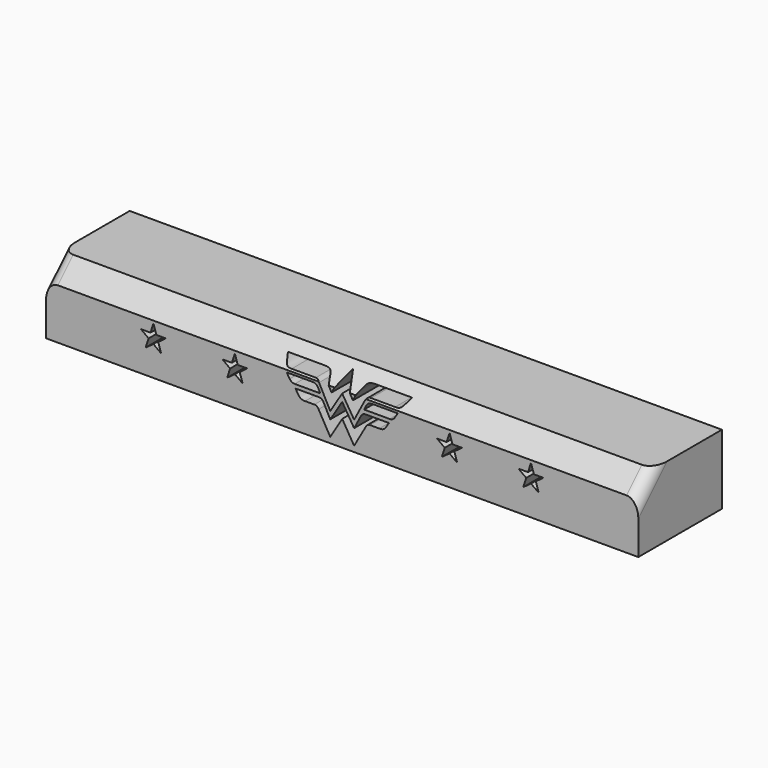
from build123d import *

# Parameters (mm, degrees)
F0_W        = 215.9
F0_H        = 25.4
F1_DEPTH    = 38.1
F3_DEPTH    = 38.1
F4_T1_DEPTH = 251.8264113419
F5_R        = 4.2924717139


# Not quite as in the source:
# - a fillet or chamfer that OpenCascade refuses, or shapes differently, is made with other operations: its cross-section is extruded or revolved along the edge and cut away or added


with BuildPart() as f1:
    # F0 (on Front) → F1 (new body)
    with BuildSketch(Plane.XZ):
        with Locations((0.6619617343, 8.3113107191)):
            Rectangle(F0_W, F0_H)
        with BuildLine():
            add(Edge.make_bspline(
                [(-16.3802020252, 9.0824095532), (-14.8727670312, 6.4565530047), (-14.5080648363, 6.1891046353), (-12.8547474742, 6.1647910625)],
                knots=[0, 0, 0, 0, 4.576169517, 4.576169517, 4.576169517, 4.576169517], degree=3))
            Line((-16.3802020252, 9.0824095532), (-8.1136170775, 9.0824095532))
            add(Edge.make_bspline(
                [(-8.1136170775, 9.0824095532), (-7.2759063914, 9.0653235093), (-6.6012172028, 8.9528746903), (-6.0469708405, 7.769481279)],
                knots=[0, 0, 0, 0, 2.4484295624, 2.4484295624, 2.4484295624, 2.4484295624], degree=3))
            Line((-6.0469708405, 7.769481279), (-3.6874657962, 3.2825956335))
            Line((-3.6874657962, 3.2825956335), (0.6619617343, 10.3273617318))
            Line((0.6619617343, 10.3273617318), (5.0113892648, 3.2825956335))
            Line((5.0113892648, 3.2825956335), (7.3708943091, 7.769481279))
            add(Edge.make_bspline(
                [(9.4375405461, 9.0824095532), (8.59982986, 9.0653235093), (7.9251406714, 8.9528746903), (7.3708943091, 7.769481279)],
                knots=[0, 0, 0, 0, 2.4484295624, 2.4484295624, 2.4484295624, 2.4484295624], degree=3))
            Line((9.4375405461, 9.0824095532), (17.7041254938, 9.0824095532))
            add(Edge.make_bspline(
                [(17.7041254938, 9.0824095532), (16.1966904998, 6.4565530047), (15.8319883049, 6.1891046353), (14.1786709428, 6.1647910625)],
                knots=[0, 0, 0, 0, 4.576169517, 4.576169517, 4.576169517, 4.576169517], degree=3))
            Line((14.1786709428, 6.1647910625), (10.7990959659, 6.1647910625))
            add(Edge.make_bspline(
                [(10.7990959659, 6.1647910625), (9.8487436771, 6.1233234592), (9.8487436771, 5.8779818937), (9.2673460022, 5.1436247304)],
                knots=[0, 0, 0, 0, 1.840934173, 1.840934173, 1.840934173, 1.840934173], degree=3))
            Line((9.2673460022, 5.1436247304), (5.0113892648, -2.3575623054))
            Line((5.0113892648, -2.3575623054), (0.6619617343, 4.8800110817))
            Line((0.6619617343, 4.8800110817), (-3.6874657962, -2.3575623054))
            Line((-3.6874657962, -2.3575623054), (-7.9434225336, 5.1436247304))
            add(Edge.make_bspline(
                [(-9.4751724973, 6.1647910625), (-8.5248202085, 6.1233234592), (-8.5248202085, 5.8779818937), (-7.9434225336, 5.1436247304)],
                knots=[0, 0, 0, 0, 1.840934173, 1.840934173, 1.840934173, 1.840934173], degree=3))
            Line((-9.4751724973, 6.1647910625), (-12.8547474742, 6.1647910625))
        make_face(mode=Mode.SUBTRACT)
        with BuildLine():
            Line((-18.4998314541, 11.4835865716), (-19.5860914445, 13.219167863))
            Line((-19.5860914445, 13.219167863), (-10.0794029066, 13.219167863))
            ThreePointArc((-10.0794029066, 13.219167863), (-8.9329270461, 12.8954335527), (-8.1251045992, 12.0198573444))
            Line((-8.1251045992, 12.0198573444), (-7.3300511576, 10.4545447975))
            Line((-7.3300511576, 10.4545447975), (-16.641804624, 10.4545447975))
            ThreePointArc((-16.641804624, 10.4545447975), (-17.7037828104, 10.7289859143), (-18.4998314541, 11.4835865716))
        make_face(mode=Mode.SUBTRACT)
        with BuildLine():
            add(Edge.make_bspline(
                [(-21.9861995429, 17.5955053419), (-19.9910327792, 14.315311797), (-19.9910327792, 14.6534768865), (-18.1987602264, 14.5858433098)],
                knots=[0, 0, 0, 0, 4.83764014, 4.83764014, 4.83764014, 4.83764014], degree=3))
            Line((-21.9861995429, 17.5955053419), (-8.4934448823, 17.5955053419))
            add(Edge.make_bspline(
                [(-8.4934448823, 17.5955053419), (-6.0586617328, 17.5616890192), (-5.8219470084, 17.1220749617), (-5.0103529356, 15.4312541708)],
                knots=[0, 0, 0, 0, 4.1007209903, 4.1007209903, 4.1007209903, 4.1007209903], degree=3))
            Line((-5.0103529356, 15.4312541708), (-3.2304712382, 12.0465927742))
            Line((-3.2304712382, 12.0465927742), (0.6619617343, 18.9819801599))
            Line((0.6619617343, 18.9819801599), (4.5543947068, 12.0465927742))
            Line((4.5543947068, 12.0465927742), (6.3342764042, 15.4312541708))
            add(Edge.make_bspline(
                [(9.8173683509, 17.5955053419), (7.3825852014, 17.5616890192), (7.145870477, 17.1220749617), (6.3342764042, 15.4312541708)],
                knots=[0, 0, 0, 0, 4.1007209903, 4.1007209903, 4.1007209903, 4.1007209903], degree=3))
            Line((9.8173683509, 17.5955053419), (23.3101230115, 17.5955053419))
            add(Edge.make_bspline(
                [(23.3101230115, 17.5955053419), (21.3149562478, 14.315311797), (21.3149562478, 14.6534768865), (19.522683695, 14.5858433098)],
                knots=[0, 0, 0, 0, 4.83764014, 4.83764014, 4.83764014, 4.83764014], degree=3))
            Line((19.522683695, 14.5858433098), (10.7304118574, 14.5858433098))
            add(Edge.make_bspline(
                [(10.7304118574, 14.5858433098), (9.9142082036, 14.5666254684), (9.6125975251, 14.456034638), (9.1072237119, 13.7742487714)],
                knots=[0, 0, 0, 0, 1.814779725, 1.814779725, 1.814779725, 1.814779725], degree=3))
            Line((9.1072237119, 13.7742487714), (5.0113892648, 5.9855217114))
            Line((5.0113892648, 5.9855217114), (0.6619617343, 13.0302878097))
            Line((0.6619617343, 13.0302878097), (-3.6874657962, 5.9855217114))
            Line((-3.6874657962, 5.9855217114), (-7.7833002433, 13.7742487714))
            add(Edge.make_bspline(
                [(-9.4064883888, 14.5858433098), (-8.590284735, 14.5666254684), (-8.2886740565, 14.456034638), (-7.7833002433, 13.7742487714)],
                knots=[0, 0, 0, 0, 1.814779725, 1.814779725, 1.814779725, 1.814779725], degree=3))
            Line((-9.4064883888, 14.5858433098), (-18.1987602264, 14.5858433098))
        make_face(mode=Mode.SUBTRACT)
        with BuildLine():
            Line((11.4033263752, 13.219167863), (20.910014913, 13.219167863))
            Line((20.910014913, 13.219167863), (19.8237549226, 11.4835865716))
            ThreePointArc((19.8237549226, 11.4835865716), (19.027706279, 10.7289859143), (17.9657280925, 10.4545447975))
            Line((17.9657280925, 10.4545447975), (8.6539746262, 10.4545447975))
            Line((8.6539746262, 10.4545447975), (9.4490280678, 12.0198573444))
            ThreePointArc((9.4490280678, 12.0198573444), (10.2568505147, 12.8954335527), (11.4033263752, 13.219167863))
        make_face(mode=Mode.SUBTRACT)
    extrude(amount=F1_DEPTH)

    # F2 (on Front) → F3 (cut, through all)
    with BuildSketch(Plane.XZ):
        Polygon((-40.2027384589, 7.7412761245), (-41.2695823308, 4.4282208097), (-38.459122454, 6.4814637683), (-35.6378924948, 4.4430445564), (-36.7221627261, 7.7504377039), (-33.9117028493, 9.8036806625), (-37.3922785821, 9.7945190831), (-38.4765488134, 13.1019122305), (-39.5433926854, 9.7888569157), (-43.0239684182, 9.7796953364), align=None)
        Polygon((39.800472282, 13.1019122305), (38.7162020507, 9.7945190831), (35.2356263179, 9.8036806625), (38.0460861947, 7.7504377039), (36.9618159633, 4.4430445564), (39.7830459226, 6.4814637683), (42.5935057994, 4.4282208097), (41.5266619275, 7.7412761245), (44.3478918867, 9.7796953364), (40.867316154, 9.7888569157), align=None)
        Polygon((-63.6021081133, 9.7796953364), (-67.082683846, 9.7888569157), (-68.149527718, 13.1019122305), (-69.2337979493, 9.7945190831), (-72.7143736821, 9.8036806625), (-69.9039138053, 7.7504377039), (-70.9881840367, 4.4430445564), (-68.1669540774, 6.4814637683), (-65.3564942006, 4.4282208097), (-66.4233380725, 7.7412761245), align=None)
        Polygon((70.5577214179, 9.7945190831), (69.4734511866, 13.1019122305), (68.4066073146, 9.7888569157), (64.9260315818, 9.7796953364), (67.7472615411, 7.7412761245), (66.6804176692, 4.4282208097), (69.490877546, 6.4814637683), (72.3121075052, 4.4430445564), (71.2278372739, 7.7504377039), (74.0382971507, 9.8036806625), align=None)
    extrude(amount=F3_DEPTH, mode=Mode.SUBTRACT)

    # F4: chamfer of 6.985 on 1 edges, made by hand

    # F4_s2 → F4_t1 (cut)
    with BuildSketch(Plane.YZ.offset(-125.2512439366)):
        Polygon((-31.115, 21.0113107191), (-38.1, 14.0263107191), (-38.1, 21.0113107191), align=None)
    extrude(amount=F4_T1_DEPTH, mode=Mode.SUBTRACT)

    # F5
    f5_edges = [f1.edges().sort_by_distance(p)[0] for p in [
        (108.611962, -34.6075, 17.518811),
        (-107.288038, -34.6075, 17.518811),
    ]]
    fillet(f5_edges, radius=F5_R)


solid = f1.part
